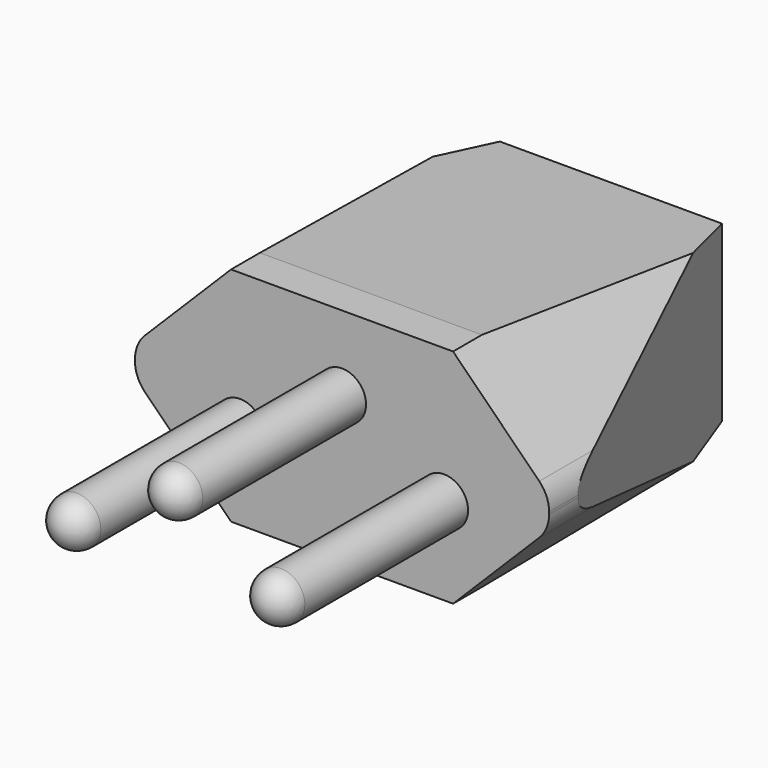
from build123d import *

# Parameters (mm, degrees)
F0_W       = 34.5
F0_H       = 18.5
F1_DEPTH   = 28
F2_R       = 2
F3_DEPTH   = 19
F4_SIZE    = 8
F5_SIZE2   = 8
F5_SIZE    = 25
F5_2_SIZE2 = 8
F5_2_SIZE  = 25
F6_SIZE2   = 2
F6_SIZE    = 25
F6_2_SIZE2 = 2
F6_2_SIZE  = 25
F7_R       = 2
F8_R       = 2.8


with BuildPart() as f1:
    # F0 (on Front) → F1 (new body)
    with BuildSketch(Plane.XZ):
        Rectangle(F0_W, F0_H)
    extrude(amount=-F1_DEPTH)

    # F2 (on face) → F3 (join)
    with BuildSketch(Plane.XZ):
        with Locations((-8.5, -2)):
            Circle(F2_R)
        with Locations((8.5, -2)):
            Circle(F2_R)
        with Locations((0, 3)):
            Circle(F2_R)
    extrude(amount=F3_DEPTH)

    # F4
    f4_edges = [f1.edges().sort_by_distance(p)[0] for p in [
        (17.25, 14, 9.25),
        (-17.25, 14, 9.25),
        (17.25, 14, -9.25),
        (-17.25, 14, -9.25),
    ]]
    chamfer(f4_edges, length=F4_SIZE)

    # F5
    f5_edges = [f1.edges().sort_by_distance(p)[0] for p in [
        (17.25, 28, 0),
    ]]
    f5_side = f1.faces().sort_by_distance((17.25, 14, 0))[0]
    chamfer(f5_edges, length=F5_SIZE, length2=F5_SIZE2, reference=f5_side)

    # F5#2
    f5_2_edges = [f1.edges().sort_by_distance(p)[0] for p in [
        (-17.25, 28, 0),
    ]]
    f5_2_side = f1.faces().sort_by_distance((-17.25, 14, 0))[0]
    chamfer(f5_2_edges, length=F5_2_SIZE, length2=F5_2_SIZE2, reference=f5_2_side)

    # F6
    f6_edges = [f1.edges().sort_by_distance(p)[0] for p in [
        (0, 28, 9.25),
    ]]
    f6_side = f1.faces().sort_by_distance((0, 14, 9.25))[0]
    chamfer(f6_edges, length=F6_SIZE, length2=F6_SIZE2, reference=f6_side)

    # F6#2
    f6_2_edges = [f1.edges().sort_by_distance(p)[0] for p in [
        (0, 28, -9.25),
    ]]
    f6_2_side = f1.faces().sort_by_distance((0, 14, -9.25))[0]
    chamfer(f6_2_edges, length=F6_2_SIZE, length2=F6_2_SIZE2, reference=f6_2_side)

    # F7
    f7_edges = [f1.edges().sort_by_distance(p)[0] for p in [
        (-10.5, -19, -2),
        (6.5, -19, -2),
        (-2, -19, 3),
    ]]
    fillet(f7_edges, radius=F7_R)

    # F8
    f8_edges = [f1.edges().sort_by_distance(p)[0] for p in [
        (-17.25, 1.5, 1.25),
        (-17.25, 1.5, -1.25),
        (17.25, 1.5, 1.25),
        (17.25, 1.5, -1.25),
    ]]
    fillet(f8_edges, radius=F8_R)


solid = f1.part
